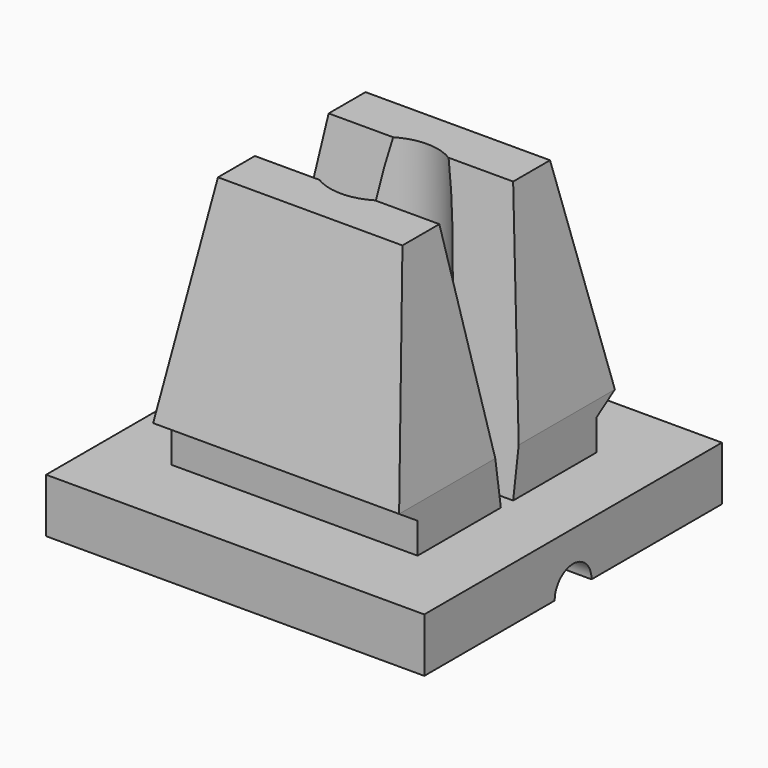
from build123d import *

# Parameters (mm, degrees)
F0_W      = 12.3
F0_H      = 12.1
F1_DEPTH  = 1.76
F2_W      = 8
F2_H      = 0.45
F2_H_2    = 7.8699186992
F3_DEPTH  = 8.3
F5_DEPTH  = 10.151
F7_DEPTH  = 12.101
F9_DEPTH  = 12.301
F11_DEPTH = 10.061


with BuildPart() as f1:
    # F0 (on Top) → F1 (new body)
    with BuildSketch(Plane.XY):
        with Locations((-6.15, 6.05)):
            Rectangle(F0_W, F0_H)
    extrude(amount=F1_DEPTH)

    # F2 (on face) → F3 (join)
    with BuildSketch(Plane.XY.offset(1.76)):
        with Locations((-6.15, 10.2099593496)):
            Rectangle(F2_W, F2_H)
        with Locations((-6.15, 6.05)):
            Rectangle(F2_W, F2_H_2)
        with Locations((-6.15, 1.8900406504)):
            Rectangle(F2_W, F2_H)
    extrude(amount=F3_DEPTH)

    # F4 (on face) → F5 (cut, through all)
    with BuildSketch(Plane(origin=(-10.15, 0, 0), x_dir=(0, -1, 0), z_dir=(-1, 0, 0))):
        Polygon((-10.4349593496, 3.26), (-9.05, 10.06), (-10.4349593496, 10.06), align=None)
        Polygon((-4.55, 10.06), (-7.55, 10.06), (-6.3, 1.76), (-5.8, 1.76), align=None)
        Polygon((-1.6650406504, 10.06), (-3.05, 10.06), (-1.6650406504, 3.26), align=None)
        Polygon((-10.4349593496, 1.76), (-9.6849593496, 1.76), (-9.6849593496, 2.76), (-10.4349593496, 3.26), align=None)
        Polygon((-2.4150406504, 2.76), (-2.4150406504, 1.76), (-1.6650406504, 1.76), (-1.6650406504, 3.26), align=None)
    extrude(amount=-F5_DEPTH, mode=Mode.SUBTRACT)

    # F6 (on Front) → F7 (cut, through all)
    with BuildSketch(Plane.XZ):
        Polygon((-10.15, 10.06), (-10.15, 3.26), (-9.15, 10.06), align=None)
        Polygon((-3.15, 10.06), (-2.15, 3.26), (-2.15, 10.06), align=None)
    extrude(amount=-F7_DEPTH, mode=Mode.SUBTRACT)

    # F8 (on face) → F9 (cut, through all)
    with BuildSketch(Plane(origin=(-12.3, 0, 0), x_dir=(0, -1, 0), z_dir=(-1, 0, 0))):
        with BuildLine():
            ThreePointArc((-6.8, 0), (-6.05, -0.75), (-5.3, 0))
            Line((-5.3, 0), (-6.8, 0))
        make_face()
        with BuildLine():
            Line((-6.8, 0), (-5.3, 0))
            ThreePointArc((-5.3, 0), (-6.05, 0.75), (-6.8, 0))
        make_face()
    extrude(amount=-F9_DEPTH, mode=Mode.SUBTRACT)

    # F10 (on face) → F11 (cut, through all)
    with BuildSketch(Plane(origin=(0, 0, 0), x_dir=(1, 0, 0), z_dir=(0, 0, -1))):
        with BuildLine():
            ThreePointArc((-7.7311388301, -5.3), (-6.5343872054, -7.7572628609), (-4.4, -6.05))
            ThreePointArc((-4.4, -6.05), (-4.4427371391, -5.6656127946), (-4.5688611699, -5.3))
            Line((-4.5688611699, -5.3), (-7.7311388301, -5.3))
        make_face()
        with BuildLine():
            Line((-7.7311388301, -5.3), (-4.5688611699, -5.3))
            ThreePointArc((-4.5688611699, -5.3), (-6.15, -4.3), (-7.7311388301, -5.3))
        make_face()
    extrude(amount=-F11_DEPTH, mode=Mode.SUBTRACT)


solid = f1.part
